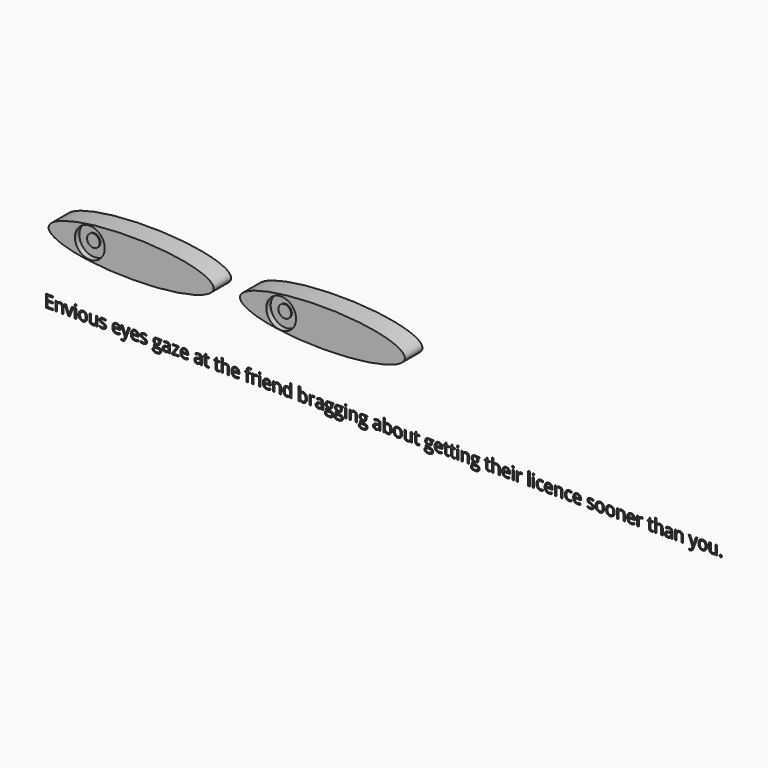
from build123d import *

# Parameters (mm, degrees)
F0_R         = 3.4334979869
F1_DEPTH     = 5.08
F0_R_2       = 1.4444034573
F2_DEPTH     = 3.81
F3_DEPTH     = 4.064
F4_TEXT_SIZE = 3.9775089438
F5_DEPTH     = 0.0508


# Not quite as in the source:
# - Text() gives the source's letters only with a copy of the font that has no kerning and outlines rounded to 1/6400 em; it was checked with that copy


with BuildPart() as f1:
    # F0 (on Front) → F1 (new body)
    with BuildSketch(Plane.XZ):
        with BuildLine():
            add(Edge.make_bspline(
                [(-17.5137091428, 16.9606450945), (-17.5137091428, 24.3979773752), (-45.9965309128, 20.6793112348), (-74.4793526828, 16.9606450945), (-45.9965309128, 13.2419789542), (-17.5137091428, 9.5233128139), (-17.5137091428, 16.9606450945)],
                knots=[0, 0, 0, 2.0943951024, 2.0943951024, 4.1887902048, 4.1887902048, 6.2831853072, 6.2831853072, 6.2831853072], degree=2, weights=[1, 0.5, 1, 0.5, 1, 0.5, 1]))
        make_face()
        with Locations((-45.9965309128, 16.9606450945)):
            Circle(F0_R, mode=Mode.SUBTRACT)
    extrude(amount=F1_DEPTH)


with BuildPart() as f1b:
    # F0 (on Front) → F1, piece 2 (new body)
    with BuildSketch(Plane.XZ):
        with BuildLine():
            add(Edge.make_bspline(
                [(26.545047426, 17.1450003982), (26.545047426, 24.5800016947), (-1.934702574, 20.8625010464), (-30.414452574, 17.1450003982), (-1.934702574, 13.4274997499), (26.545047426, 9.7099991016), (26.545047426, 17.1450003982)],
                knots=[0, 0, 0, 2.0943951024, 2.0943951024, 4.1887902048, 4.1887902048, 6.2831853072, 6.2831853072, 6.2831853072], degree=2, weights=[1, 0.5, 1, 0.5, 1, 0.5, 1]))
        make_face()
        with Locations((-1.934702574, 16.9606450945)):
            Circle(F0_R, mode=Mode.SUBTRACT)
    extrude(amount=F1_DEPTH)


with BuildPart() as f2:
    # F0 (on Front) → F2 (new body)
    with BuildSketch(Plane.XZ):
        with Locations((-45.9965309128, 16.9606450945)):
            Circle(F0_R)
        with Locations((-45.9965309128, 16.9606450945)):
            Circle(F0_R_2, mode=Mode.SUBTRACT)
    extrude(amount=F2_DEPTH)


with BuildPart() as f2b:
    # F0 (on Front) → F2, piece 2 (new body)
    with BuildSketch(Plane.XZ):
        with Locations((-1.934702574, 16.9606450945)):
            Circle(F0_R)
        with Locations((-1.934702574, 16.9606450945)):
            Circle(F0_R_2, mode=Mode.SUBTRACT)
    extrude(amount=F2_DEPTH)


with BuildPart() as f3:
    # F0 (on Front) → F3 (new body)
    with BuildSketch(Plane.XZ):
        with Locations((-45.9965309128, 16.9606450945)):
            Circle(F0_R_2)
    extrude(amount=F3_DEPTH)


with BuildPart() as f3b:
    # F0 (on Front) → F3, piece 2 (new body)
    with BuildSketch(Plane.XZ):
        with Locations((-1.934702574, 16.9606450945)):
            Circle(F0_R_2)
    extrude(amount=F3_DEPTH)


with BuildPart() as f5:
    # F4 (on Front) → F5 (new body)
    with BuildSketch(Plane.XZ):
        with Locations((-60.4830160737, -2.8638064396)):
            Text('Envious eyes gaze at the friend bragging about getting their licence sooner than you.', F4_TEXT_SIZE, font='Open Sans', text_align=(TextAlign.LEFT, TextAlign.BOTTOM))
    extrude(amount=F5_DEPTH)


solid = Compound([f1.part, f1b.part, f2.part, f2b.part, f3.part, f3b.part, f5.part])
